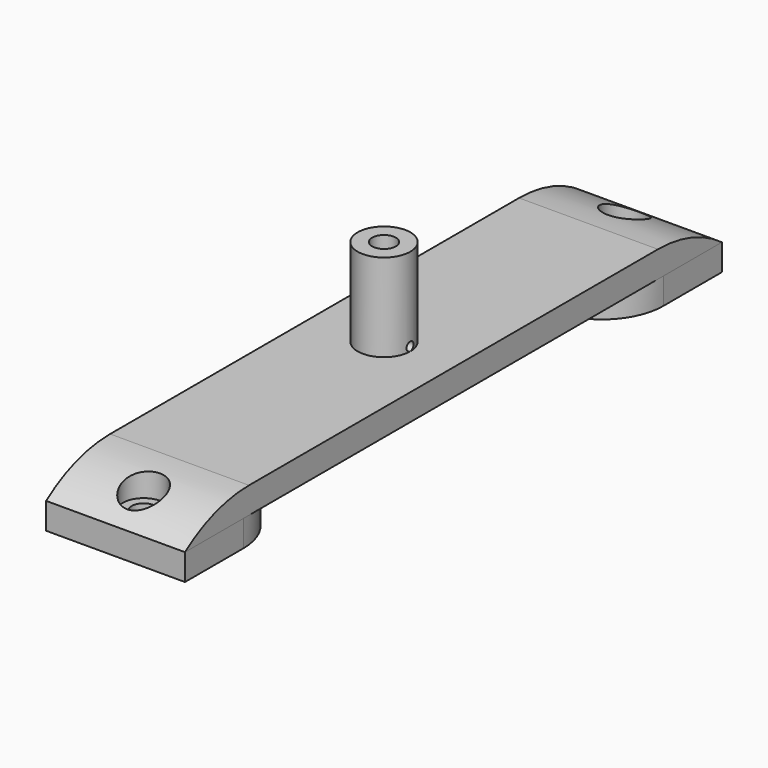
from build123d import *

# Parameters (mm, degrees)
F0_W              = 15.83
F0_H              = 15.33
F1_DEPTH          = 3
F2_R              = 7
F2_2_R            = 7
F5_W              = 15.83
F5_H              = 76.5
F6_DEPTH          = 3
F7_T1_DEPTH       = 61.4260524607
F11_D             = 2.7
F11_DEPTH         = 10
F11_CBORE_D       = 4.7
F11_CBORE_DEPTH   = 3
F11_TIP           = 0.8111618357
F11_2_D           = 2.7
F11_2_DEPTH       = 10
F11_2_CBORE_D     = 4.7
F11_2_CBORE_DEPTH = 3
F11_2_TIP         = 0.8111618357
F11_3_D           = 2.7
F11_3_DEPTH       = 10
F11_3_CBORE_D     = 4.7
F11_3_CBORE_DEPTH = 3
F11_3_TIP         = 0.8111618357
F12_R             = 3
F13_DEPTH         = 10
F15_D             = 2.7
F15_DEPTH         = 20
F15_TIP           = 0.8111618357
F17_D             = 1


# Not quite as in the source:
# - a fillet or chamfer that OpenCascade refuses, or shapes differently, is made with other operations: its cross-section is extruded or revolved along the edge and cut away or added


with BuildPart() as f1:
    # F0 (on Top) → F1 (new body)
    with BuildSketch(Plane.XY):
        with Locations((0, 30.585)):
            Rectangle(F0_W, F0_H)
    extrude(amount=F1_DEPTH)

    # F2
    f2_edges = [f1.edges().sort_by_distance(p)[0] for p in [
        (-7.915, 22.92, 1.5),
        (7.915, 22.92, 1.5),
    ]]
    fillet(f2_edges, radius=F2_R)

    # F11
    with Locations(Plane.XY.offset(6)):
        with Locations((0, 34.25), (0, -34.25)):
            CounterBoreHole(F11_D / 2, F11_CBORE_D / 2, F11_CBORE_DEPTH, depth=F11_DEPTH)
            with Locations((0, 0, -(F11_DEPTH + F11_TIP / 2))):  # 118° drill point
                Cone(0, F11_D / 2, F11_TIP, mode=Mode.SUBTRACT)


with BuildPart() as f1b:
    # F0 (on Top) → F1, piece 2 (new body)
    with BuildSketch(Plane.XY):
        with Locations((0, -30.585)):
            Rectangle(F0_W, F0_H)
    extrude(amount=F1_DEPTH)

    # F2#2
    f2_2_edges = [f1b.edges().sort_by_distance(p)[0] for p in [
        (-7.915, -22.92, 1.5),
        (7.915, -22.92, 1.5),
    ]]
    fillet(f2_2_edges, radius=F2_2_R)

    # F11#2
    with Locations(Plane.XY.offset(6)):
        with Locations((0, 34.25), (0, -34.25)):
            CounterBoreHole(F11_2_D / 2, F11_2_CBORE_D / 2, F11_2_CBORE_DEPTH, depth=F11_2_DEPTH)
            with Locations((0, 0, -(F11_2_DEPTH + F11_2_TIP / 2))):  # 118° drill point
                Cone(0, F11_2_D / 2, F11_2_TIP, mode=Mode.SUBTRACT)


with BuildPart() as f6:
    # F5 (on face) → F6 (new body)
    with BuildSketch(Plane(origin=(0, 0, 3), x_dir=(1, 0, 0), z_dir=(0, 0, -1))):
        Rectangle(F5_W, F5_H)
    extrude(amount=-F6_DEPTH)

    # F7: fillet of radius 15.36 on 2 edges, made by hand

    # F7_s2 → F7_t1 (cut)
    with BuildSketch(Plane.YZ.offset(-30.7130262304)):
        with BuildLine():
            ThreePointArc((38.25, 3), (33.9307895079, 5.2307367874), (29.1307895079, 6))
            Line((29.1307895079, 6), (38.25, 6))
            Line((38.25, 6), (38.25, 3))
        make_face()
        with BuildLine():
            ThreePointArc((-38.25, 3), (-33.9307895079, 5.2307367874), (-29.1307895079, 6))
            Line((-29.1307895079, 6), (-38.25, 6))
            Line((-38.25, 6), (-38.25, 3))
        make_face()
    extrude(amount=F7_T1_DEPTH, mode=Mode.SUBTRACT)

    # F11#3
    with Locations(Plane.XY.offset(6)):
        with Locations((0, 34.25), (0, -34.25)):
            CounterBoreHole(F11_3_D / 2, F11_3_CBORE_D / 2, F11_3_CBORE_DEPTH, depth=F11_3_DEPTH)
            with Locations((0, 0, -(F11_3_DEPTH + F11_3_TIP / 2))):  # 118° drill point
                Cone(0, F11_3_D / 2, F11_3_TIP, mode=Mode.SUBTRACT)

    # F12 (on face) → F13 (join)
    with BuildSketch(Plane.XY.offset(6)):
        Circle(F12_R)
    extrude(amount=F13_DEPTH)

    # F15
    with Locations(Plane.XY.offset(16)):
        with Locations((0, 0)):
            Hole(F15_D / 2, depth=F15_DEPTH)
            with Locations((0, 0, -(F15_DEPTH + F15_TIP / 2))):  # 118° drill point
                Cone(0, F15_D / 2, F15_TIP, mode=Mode.SUBTRACT)

    # F17 (through all)
    with Locations(Plane.YZ.offset(7.915)):
        with Locations((0, 6.5)):
            Hole(F17_D / 2)


solid = Compound([f1.part, f1b.part, f6.part])
